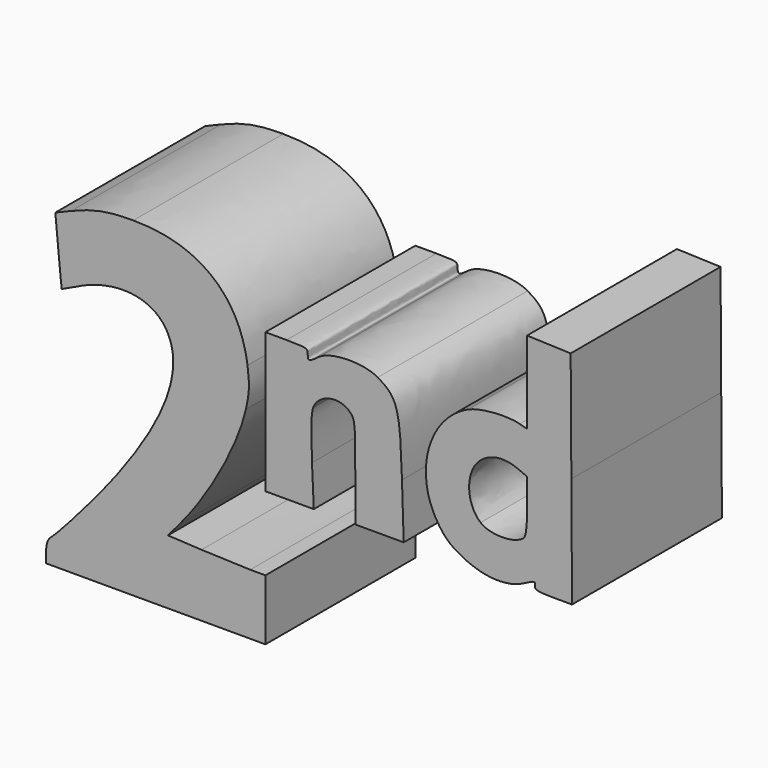
from build123d import *

# Parameters (mm, degrees)
F1_DEPTH = 6.35


# Not quite as in the source:
# - ends of sketch curves that miss each other by under 0.0002 mm in the source are joined


with BuildPart() as f1:
    # F0 (on Front) → F1 (new body)
    with BuildSketch(Plane.XZ):
        with BuildLine():
            add(Edge.make_bspline(
                [(-8.9133755493, -5.7023881004), (-8.9133755493, -5.4868837545), (-8.8566497364, -5.3084137598), (-8.7639088993, -5.2321362172)],
                knots=[0, 0, 0, 0, 1, 1, 1, 1], degree=3))
            Line((-8.9133755493, -5.7023881004), (-8.9133755493, -6.0497027056))
            Line((-8.9133755493, -6.0497027056), (-5.196146377, -6.0497027056))
            Line((-5.196146377, -6.0497027056), (-1.4789172047, -6.0497027056))
            Line((-1.4789172047, -6.0497027056), (-1.4789172047, -5.0196271518))
            Line((-1.4789172047, -5.0196271518), (-1.4789172047, -3.9895515981))
            Line((-1.4789172047, -3.9895515981), (-1.9939549816, -3.9891933109))
            add(Edge.make_bspline(
                [(-3.6463520247, -3.9308220643), (-3.0208050553, -3.9627266392), (-2.2772257589, -3.9889935658), (-1.9939549816, -3.9891933109)],
                knots=[0, 0, 0, 0, 1, 1, 1, 1], degree=3))
            Line((-3.6463520247, -3.9308220643), (-4.7837121867, -3.8728135834))
            Line((-4.7837121867, -3.8728135834), (-4.3970773583, -3.4161479489))
            add(Edge.make_bspline(
                [(-2.1407595581, 0.7483248017), (-2.4010757734, -0.4154115645), (-3.3689284937, -2.2017703813), (-4.3970773583, -3.4161479489)],
                knots=[0, 0, 0, 0, 1, 1, 1, 1], degree=3))
            add(Edge.make_bspline(
                [(-2.0863554459, 2.0788707074), (-2.0094715023, 1.5309663546), (-2.0192652815, 1.2914603526), (-2.1407595581, 0.7483248017)],
                knots=[0, 0, 0, 0, 1, 1, 1, 1], degree=3))
            add(Edge.make_bspline(
                [(-5.9539326546, 5.1445753005), (-3.749439299, 5.1508811543), (-2.3632442333, 4.0520932911), (-2.0863554459, 2.0788707074)],
                knots=[0, 0, 0, 0, 1, 1, 1, 1], degree=3))
            add(Edge.make_bspline(
                [(-8.0628135016, 4.7419178708), (-7.318555251, 5.0513462971), (-6.8436142847, 5.1420287746), (-5.9539326546, 5.1445753005)],
                knots=[0, 0, 0, 0, 1, 1, 1, 1], degree=3))
            Line((-8.0628135016, 4.7419178708), (-8.6006141568, 4.5183251925))
            Line((-8.6006141568, 4.5183251925), (-8.4965111385, 3.4217900597))
            add(Edge.make_bspline(
                [(-8.3841755772, 2.3100098088), (-8.3886989524, 2.318393728), (-8.4392541649, 2.8186951545), (-8.4965111385, 3.4217900597)],
                knots=[0, 0, 0, 0, 1, 1, 1, 1], degree=3))
            add(Edge.make_bspline(
                [(-7.8535836594, 2.5557930016), (-8.14088248, 2.4122282367), (-8.379648619, 2.3016258895), (-8.3841755772, 2.3100098088)],
                knots=[0, 0, 0, 0, 1, 1, 1, 1], degree=3))
            add(Edge.make_bspline(
                [(-4.8147631425, 2.2103388025), (-5.2902934912, 3.056431218), (-6.562335584, 3.2010377028), (-7.8535836594, 2.5557930016)],
                knots=[0, 0, 0, 0, 1, 1, 1, 1], degree=3))
            add(Edge.make_bspline(
                [(-6.496803073, -2.6036763037), (-4.8035326318, -0.3508383673), (-4.2560107506, 1.2161734739), (-4.8147631425, 2.2103388025)],
                knots=[0, 0, 0, 0, 1, 1, 1, 1], degree=3))
            add(Edge.make_bspline(
                [(-8.7639088993, -5.2321362172), (-8.4579039067, -4.9804556178), (-7.0994528064, -3.4054817404), (-6.496803073, -2.6036763037)],
                knots=[0, 0, 0, 0, 1, 1, 1, 1], degree=3))
        make_face()
    extrude(amount=F1_DEPTH)


with BuildPart() as f1b:
    # F0 (on Front) → F1, piece 2 (new body)
    with BuildSketch(Plane.XZ):
        with BuildLine():
            add(Edge.make_bspline(
                [(5.247696732, -1.2926256975), (4.814993342, -1.0764011944), (4.6218004326, -0.9108411814), (4.3836586089, -0.5521733522)],
                knots=[0, 0, 0, 0, 1, 1, 1, 1], degree=3))
            add(Edge.make_bspline(
                [(7.2543322795, -1.3919751411), (6.6989639097, -1.6751178307), (5.9377067253, -1.6374278141), (5.247696732, -1.2926256975)],
                knots=[0, 0, 0, 0, 1, 1, 1, 1], degree=3))
            add(Edge.make_bspline(
                [(7.6574053223, -1.3471892475), (7.6574053223, -1.1796102863), (7.6746272899, -1.177697033), (7.2543322795, -1.3919751411)],
                knots=[0, 0, 0, 0, 1, 1, 1, 1], degree=3))
            add(Edge.make_bspline(
                [(8.2853904358, -1.4815469284), (7.7868956723, -1.4815469284), (7.6574053223, -1.4538423746), (7.6574053223, -1.3471892475)],
                knots=[0, 0, 0, 0, 1, 1, 1, 1], degree=3))
            Line((8.2853904358, -1.4815469284), (8.9133755493, -1.4815469284))
            Line((8.9133755493, -1.4815469284), (8.89, 2.2580751908))
            Line((8.89, 2.2580751908), (8.8666244507, 5.9976976458))
            Line((8.8666244507, 5.9976976458), (8.1276572056, 6.0237128757))
            Line((8.1276572056, 6.0237128757), (7.3886899605, 6.0497281056))
            Line((7.3886899605, 6.0497281056), (7.3886899605, 4.6560364412))
            Line((7.3886899605, 4.6560364412), (7.3886899605, 3.2623451126))
            Line((7.3886899605, 3.2623451126), (7.1423675454, 3.3312302956))
            add(Edge.make_bspline(
                [(5.4051066081, 3.1994728837), (5.8193537314, 3.3827134718), (6.7152928465, 3.4506635254), (7.1423675454, 3.3312302956)],
                knots=[0, 0, 0, 0, 1, 1, 1, 1], degree=3))
            add(Edge.make_bspline(
                [(4.3836586089, -0.5521733522), (3.521845225, 0.7458114174), (4.0234991855, 2.5883218919), (5.4051066081, 3.1994728837)],
                knots=[0, 0, 0, 0, 1, 1, 1, 1], degree=3))
        make_face()
        with BuildLine():
            add(Edge.make_bspline(
                [(7.2568716397, -0.0462907077), (7.3567182067, 0.0365739442), (7.3886899605, 0.2788091986), (7.3886899605, 0.9524293463)],
                knots=[0, 0, 0, 0, 1, 1, 1, 1], degree=3))
            add(Edge.make_bspline(
                [(5.8158299773, -0.0439546755), (6.1336315743, -0.3077077603), (6.9403079248, -0.3090146127), (7.2568716397, -0.0462907077)],
                knots=[0, 0, 0, 0, 1, 1, 1, 1], degree=3))
            add(Edge.make_bspline(
                [(5.7500197937, 1.7580003809), (5.291141736, 1.2991214275), (5.3253250172, 0.3631276005), (5.8158299773, -0.0439546755)],
                knots=[0, 0, 0, 0, 1, 1, 1, 1], degree=3))
            add(Edge.make_bspline(
                [(7.0559988453, 1.9807573545), (6.5865208623, 2.1769177772), (6.0830638217, 2.091044409), (5.7500197937, 1.7580003809)],
                knots=[0, 0, 0, 0, 1, 1, 1, 1], degree=3))
            Line((7.0559988453, 1.9807573545), (7.3886899605, 1.8417500021))
            Line((7.3886899605, 1.8417500021), (7.3886899605, 0.9524293463))
        make_face(mode=Mode.SUBTRACT)
    extrude(amount=F1_DEPTH)


with BuildPart() as f1c:
    # F0 (on Front) → F1, piece 3 (new body)
    with BuildSketch(Plane.XZ):
        with BuildLine():
            add(Edge.make_bspline(
                [(-0.7623429064, 3.2657577977), (-0.1054834315, 3.2657577977), (-0.0457686081, 3.2508288679), (-0.0457686081, 3.0866142232)],
                knots=[0, 0, 0, 0, 1, 1, 1, 1], degree=3))
            Line((-0.7623429064, 3.2657577977), (-1.4789172047, 3.2657577977))
            Line((-1.4789172047, 3.2657577977), (-1.4789172047, 0.8921054347))
            Line((-1.4789172047, 0.8921054347), (-1.4789172047, -1.4815469284))
            Line((-1.4789172047, -1.4815469284), (-0.6592341349, -1.4815469284))
            Line((-0.6592341349, -1.4815469284), (0.1604498306, -1.4815469284))
            Line((0.1604498306, -1.4815469284), (0.0994514435, -0.1142237426))
            add(Edge.make_bspline(
                [(0.1351583407, 1.5305086428), (0.0712811164, 1.3472698461), (0.0591602621, 0.7889438158), (0.0994514435, -0.1142237426)],
                knots=[0, 0, 0, 0, 1, 1, 1, 1], degree=3))
            add(Edge.make_bspline(
                [(1.3704903322, 1.82912038), (1.0003653757, 2.1739439938), (0.3004854671, 2.0047652806), (0.1351583407, 1.5305086428)],
                knots=[0, 0, 0, 0, 1, 1, 1, 1], degree=3))
            add(Edge.make_bspline(
                [(1.566523563, 0.082470528), (1.566523563, 1.576057688), (1.557700742, 1.6547115702), (1.3704903322, 1.82912038)],
                knots=[0, 0, 0, 0, 1, 1, 1, 1], degree=3))
            Line((1.566523563, 0.082470528), (1.566523563, -1.4815469284))
            Line((1.566523563, -1.4815469284), (2.3868927527, -1.4815469284))
            Line((2.3868927527, -1.4815469284), (3.2072610466, -1.4815469284))
            Line((3.2072610466, -1.4815469284), (3.1498509053, 0.3639435995))
            add(Edge.make_bspline(
                [(2.3276293711, 3.1544155875), (2.9988973636, 2.7652405033), (3.0841499993, 2.4759084031), (3.1498509053, 0.3639435995)],
                knots=[0, 0, 0, 0, 1, 1, 1, 1], degree=3))
            add(Edge.make_bspline(
                [(0.3231838537, 3.1086623186), (0.7379809478, 3.415334621), (1.8344148644, 3.4403618741), (2.3276293711, 3.1544155875)],
                knots=[0, 0, 0, 0, 1, 1, 1, 1], degree=3))
            add(Edge.make_bspline(
                [(-0.0457686081, 3.0866142232), (-0.0457686081, 2.8600692588), (-0.0101799456, 2.8621965887), (0.3231838537, 3.1086623186)],
                knots=[0, 0, 0, 0, 1, 1, 1, 1], degree=3))
        make_face()
    extrude(amount=F1_DEPTH)


solid = Compound([f1.part, f1b.part, f1c.part])
